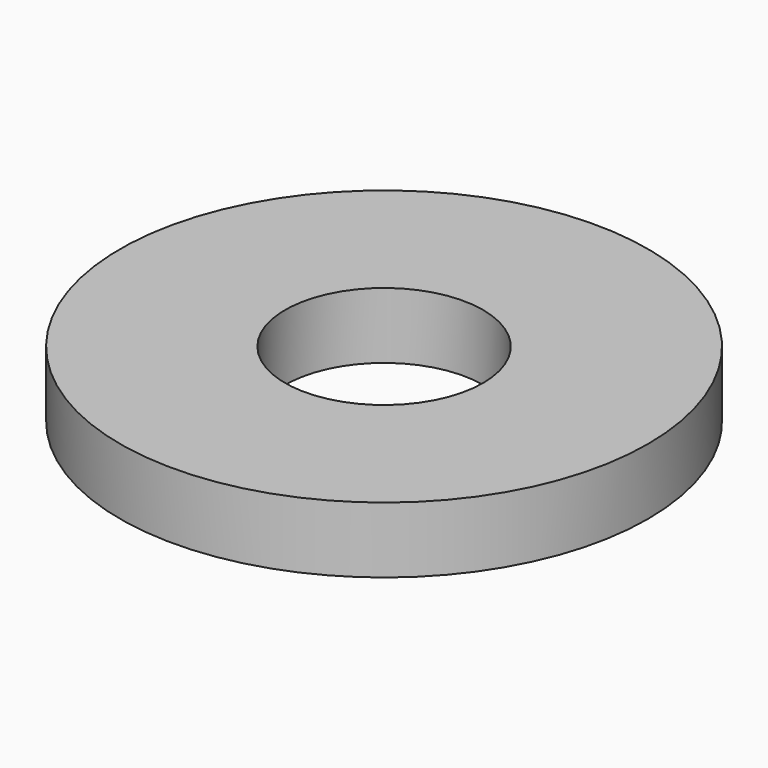
from build123d import *

# Parameters (mm, degrees)
F0_R     = 12.7
F0_R_2   = 4.7625
F1_DEPTH = 3.175


# Not quite as in the source:
# - a length typed as a fraction of an inch, garbled in the dataset ("3 / 203.2 mm" for 3/8 in), is restored


with BuildPart() as f1:
    # F0 (on Top) → F1 (new body)
    with BuildSketch(Plane.XY):
        Circle(F0_R)
        Circle(F0_R_2, mode=Mode.SUBTRACT)
    extrude(amount=F1_DEPTH)


solid = f1.part
